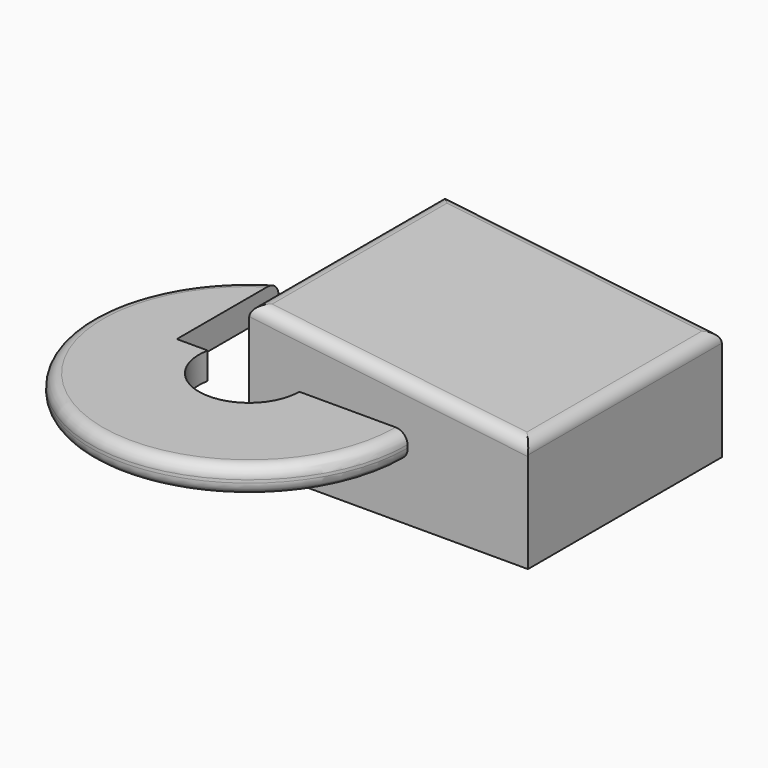
from build123d import *

# Parameters (mm, degrees)
F1_DEPTH = 102.6981025934
F4_R     = 5.08
F5_W     = 33.7471216917
F5_H     = 65.5695050955
F6_DEPTH = 25.4


with BuildPart() as f1:
    # F0 (on Front) → F1 (new body)
    with BuildSketch(Plane.XZ):
        Polygon((62.229424715, -34.6546843648), (62.229424715, 12.4018825591), (-55.8673739433, 26.1995047331), (-55.8673739433, -34.6546843648), align=None)
    extrude(amount=F1_DEPTH)

    # F2 (on face) → F3 (revolve)
    with BuildSketch(Plane.XZ.offset(102.6981025934)):
        Polygon((-34.6154049039, -11.3538783044), (11.5415975451, -11.3538783044), (11.0295861959, 0), (-34.6154049039, 0), align=None)
    revolve(axis=Axis((-55.8673739433, -102.6981025934, -4.2275898159), (0, 0, 1)))

    # F4
    f4_edges = [f1.edges().sort_by_distance(p)[0] for p in [
        (62.229425, -51.349051, 12.401883),
        (-55.867374, -51.349051, 26.199505),
        (3.181025, 0, 19.300694),
        (3.181025, -102.698103, 19.300694),
        (-103.532715, -150.363443, -11.353878),
        (-103.170668, -150.001397, 0),
    ]]
    fillet(f4_edges, radius=F4_R)

    # F5 (on Top) → F6 (cut)
    with BuildSketch(Plane.XY):
        with Locations((-72.9322209954, -65.7769069076)):
            Rectangle(F5_W, F5_H)
    extrude(amount=-F6_DEPTH, mode=Mode.SUBTRACT)


solid = f1.part
